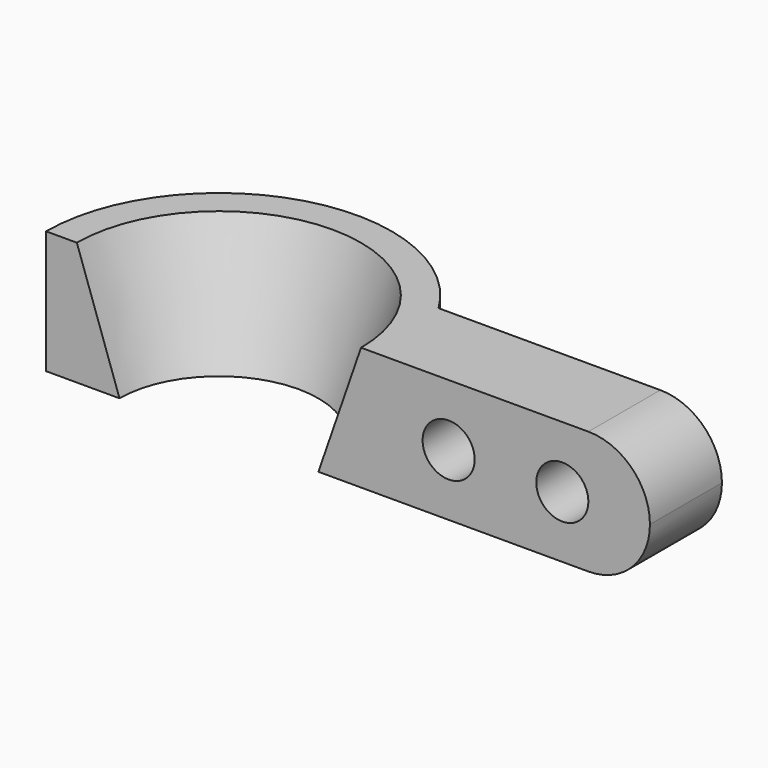
from build123d import *

# Parameters (mm, degrees)
F1_DEPTH = 52
F2_W     = 21
F2_H     = 52
F4_R     = 11
F5_DEPTH = 88.3
F6_R     = 25.99999


# Not quite as in the source:
# - a fillet or chamfer is up to 0.001 mm smaller than in the source, because OpenCascade refuses the exact size


with BuildPart() as f1:
    # F0 (on Top) → F1 (new body)
    with BuildSketch(Plane.XY):
        with BuildLine():
            Line((182, 38), (62.329768169, 38))
            ThreePointArc((62.329768169, 38), (-19.7348286497, 70.2818364741), (-73, 0))
            Line((-73, 0), (-21, 0))
            ThreePointArc((-21, 0), (0, 21), (21, 0))
            Line((21, 0), (73, 0))
            Line((73, 0), (182, 0))
            Line((182, 0), (182, 38))
        make_face()
    extrude(amount=F1_DEPTH)

    # F2 (on face) → F3 (revolve, cut)
    with BuildSketch(Plane.XZ):
        Polygon((-21, 52), (-60, 52), (-42, 0), (-21, 0), align=None)
        with Locations((-10.5, 26)):
            Rectangle(F2_W, F2_H)
    revolve(axis=Axis((0, 0, 26), (0, 0, 1)), mode=Mode.SUBTRACT)

    # F4 (on face) → F5 (cut)
    with BuildSketch(Plane.XZ):
        with Locations((97, 26)):
            Circle(F4_R)
        with Locations((145, 26)):
            Circle(F4_R)
    extrude(amount=-F5_DEPTH, mode=Mode.SUBTRACT)

    # F6 (radius 26 in the source; OpenCascade refuses exactly that, so slightly less here)
    f6_edges = [f1.edges().sort_by_distance(p)[0] for p in [
        (182, 19, 52),
        (182, 19, 0),
    ]]
    fillet(f6_edges, radius=F6_R)


solid = f1.part
